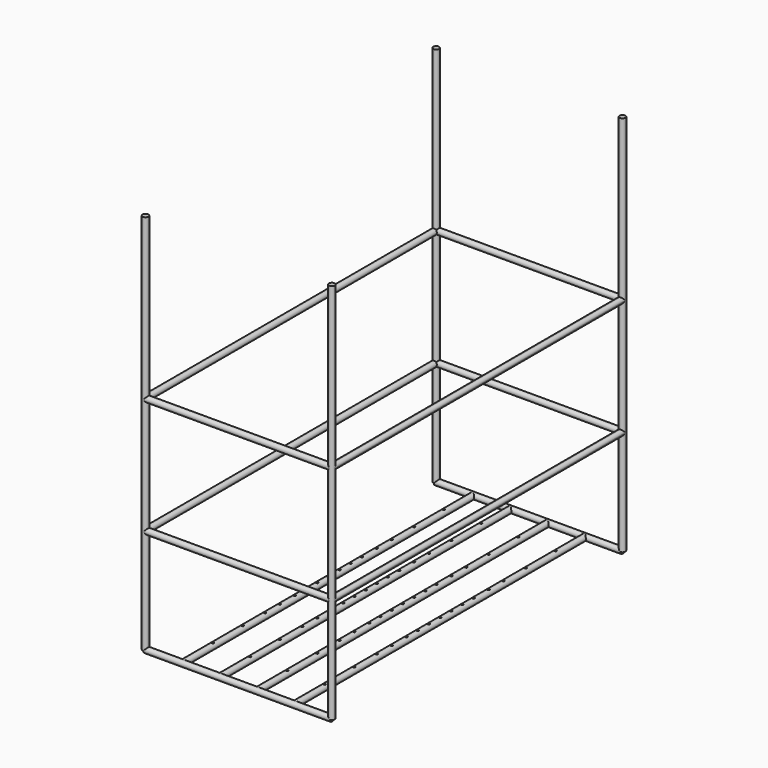
from build123d import *

# Parameters (mm, degrees)
F0_R     = 6.35
F1_DEPTH = 400
F2_R     = 6.35
F3_DEPTH = 820
F4_R     = 6.35
F4_R_2   = 5
F5_DEPTH = 780
F6_R     = 2.5
F7_DEPTH = 25


with BuildPart() as f1:
    # F0 (on Right) → F1 (new body)
    with BuildSketch(Plane.YZ):
        Circle(F0_R)
    extrude(amount=-F1_DEPTH)

    # F2 (on Top) → F3, piece 2 (join)
    with BuildSketch(Plane.XY):
        Circle(F2_R)
        with Locations((-400, 0)):
            Circle(F2_R)
    extrude(amount=F3_DEPTH)

    # F4 (on Front) → F5 (join)
    with BuildSketch(Plane.XZ):
        with BuildLine():
            ThreePointArc((0, 481.35), (-6.35, 475), (0, 468.65))
            Line((0, 468.65), (0, 475))
            Line((0, 475), (0, 481.35))
        make_face()
        with BuildLine():
            Line((0, 475), (0, 468.65))
            ThreePointArc((0, 468.65), (4.4901280605, 470.5098719395), (6.35, 475))
            ThreePointArc((6.35, 475), (4.4901280605, 479.4901280605), (0, 481.35))
            Line((0, 481.35), (0, 475))
        make_face()
        with BuildLine():
            ThreePointArc((0, 231.35), (-6.35, 225), (0, 218.65))
            Line((0, 218.65), (0, 225))
            Line((0, 225), (0, 231.35))
        make_face()
        with BuildLine():
            Line((0, 225), (0, 218.65))
            ThreePointArc((0, 218.65), (4.4901280605, 220.5098719395), (6.35, 225))
            ThreePointArc((6.35, 225), (4.4901280605, 229.4901280605), (0, 231.35))
            Line((0, 231.35), (0, 225))
        make_face()
        with Locations((-80, 0)):
            Circle(F4_R)
        with Locations((-80, 0)):
            Circle(F4_R_2, mode=Mode.SUBTRACT)
        with Locations((-400, 225)):
            Circle(F4_R)
        with Locations((-400, 475)):
            Circle(F4_R)
        with Locations((-160, 0)):
            Circle(F4_R)
        with Locations((-160, 0)):
            Circle(F4_R_2, mode=Mode.SUBTRACT)
        with Locations((-240, 0)):
            Circle(F4_R)
        with Locations((-240, 0)):
            Circle(F4_R_2, mode=Mode.SUBTRACT)
        with Locations((-320, 0)):
            Circle(F4_R)
        with Locations((-320, 0)):
            Circle(F4_R_2, mode=Mode.SUBTRACT)
    extrude(amount=-F5_DEPTH)

    # F6 (on Top) → F7 (cut)
    with BuildSketch(Plane.XY):
        with Locations((-80, 80)):
            Circle(F6_R)
        with Locations((-80, 160)):
            Circle(F6_R)
        with Locations((-80, 220)):
            Circle(F6_R)
        with Locations((-80, 300)):
            Circle(F6_R)
        with Locations((-80, 260)):
            Circle(F6_R)
        with Locations((-80, 330)):
            Circle(F6_R)
        with Locations((-80, 360)):
            Circle(F6_R)
        with Locations((-80, 420)):
            Circle(F6_R)
        with Locations((-80, 450)):
            Circle(F6_R)
        with Locations((-80, 480)):
            Circle(F6_R)
        with Locations((-80, 520)):
            Circle(F6_R)
        with Locations((-80, 560)):
            Circle(F6_R)
        with Locations((-80, 620)):
            Circle(F6_R)
        with Locations((-80, 700)):
            Circle(F6_R)
        with Locations((-80, 390)):
            Circle(F6_R)
        with Locations((-160, 560)):
            Circle(F6_R)
        with Locations((-160, 700)):
            Circle(F6_R)
        with Locations((-160, 620)):
            Circle(F6_R)
        with Locations((-160, 520)):
            Circle(F6_R)
        with Locations((-160, 420)):
            Circle(F6_R)
        with Locations((-160, 480)):
            Circle(F6_R)
        with Locations((-160, 450)):
            Circle(F6_R)
        with Locations((-160, 220)):
            Circle(F6_R)
        with Locations((-160, 390)):
            Circle(F6_R)
        with Locations((-160, 80)):
            Circle(F6_R)
        with Locations((-160, 330)):
            Circle(F6_R)
        with Locations((-160, 160)):
            Circle(F6_R)
        with Locations((-160, 360)):
            Circle(F6_R)
        with Locations((-160, 260)):
            Circle(F6_R)
        with Locations((-160, 300)):
            Circle(F6_R)
        with Locations((-240, 560)):
            Circle(F6_R)
        with Locations((-240, 700)):
            Circle(F6_R)
        with Locations((-240, 620)):
            Circle(F6_R)
        with Locations((-240, 520)):
            Circle(F6_R)
        with Locations((-240, 420)):
            Circle(F6_R)
        with Locations((-240, 480)):
            Circle(F6_R)
        with Locations((-240, 450)):
            Circle(F6_R)
        with Locations((-240, 220)):
            Circle(F6_R)
        with Locations((-240, 390)):
            Circle(F6_R)
        with Locations((-240, 80)):
            Circle(F6_R)
        with Locations((-240, 330)):
            Circle(F6_R)
        with Locations((-240, 160)):
            Circle(F6_R)
        with Locations((-240, 360)):
            Circle(F6_R)
        with Locations((-240, 260)):
            Circle(F6_R)
        with Locations((-240, 300)):
            Circle(F6_R)
        with Locations((-320, 560)):
            Circle(F6_R)
        with Locations((-320, 700)):
            Circle(F6_R)
        with Locations((-320, 620)):
            Circle(F6_R)
        with Locations((-320, 520)):
            Circle(F6_R)
        with Locations((-320, 420)):
            Circle(F6_R)
        with Locations((-320, 480)):
            Circle(F6_R)
        with Locations((-320, 450)):
            Circle(F6_R)
        with Locations((-320, 220)):
            Circle(F6_R)
        with Locations((-320, 390)):
            Circle(F6_R)
        with Locations((-320, 80)):
            Circle(F6_R)
        with Locations((-320, 330)):
            Circle(F6_R)
        with Locations((-320, 160)):
            Circle(F6_R)
        with Locations((-320, 360)):
            Circle(F6_R)
        with Locations((-320, 260)):
            Circle(F6_R)
        with Locations((-320, 300)):
            Circle(F6_R)
    extrude(amount=F7_DEPTH, mode=Mode.SUBTRACT)


with BuildPart() as f1b:
    # F0 (on Right) → F1, piece 2 (new body)
    with BuildSketch(Plane.YZ):
        with Locations((0, 225)):
            Circle(F0_R)
    extrude(amount=-F1_DEPTH)


with BuildPart() as f1c:
    # F0 (on Right) → F1, piece 3 (new body)
    with BuildSketch(Plane.YZ):
        with Locations((0, 475)):
            Circle(F0_R)
    extrude(amount=-F1_DEPTH)


with BuildPart() as f1d:
    # F0 (on Right) → F1, piece 4 (new body)
    with BuildSketch(Plane.YZ):
        with Locations((780, 0)):
            Circle(F0_R)
    extrude(amount=-F1_DEPTH)


with BuildPart() as f1e:
    # F0 (on Right) → F1, piece 5 (new body)
    with BuildSketch(Plane.YZ):
        with Locations((780, 225)):
            Circle(F0_R)
    extrude(amount=-F1_DEPTH)


with BuildPart() as f1f:
    # F0 (on Right) → F1, piece 6 (new body)
    with BuildSketch(Plane.YZ):
        with Locations((780, 475)):
            Circle(F0_R)
    extrude(amount=-F1_DEPTH)


with BuildPart() as f3:
    # F2 (on Top) → F3 (new body)
    with BuildSketch(Plane.XY):
        with Locations((0, 780)):
            Circle(F2_R)
    extrude(amount=F3_DEPTH)


with BuildPart() as f3b:
    # F2 (on Top) → F3, piece 3 (new body)
    with BuildSketch(Plane.XY):
        with Locations((-400, 780)):
            Circle(F2_R)
    extrude(amount=F3_DEPTH)


solid = Compound([f1.part, f1b.part, f1c.part, f1d.part, f1e.part, f1f.part, f3.part, f3b.part])
